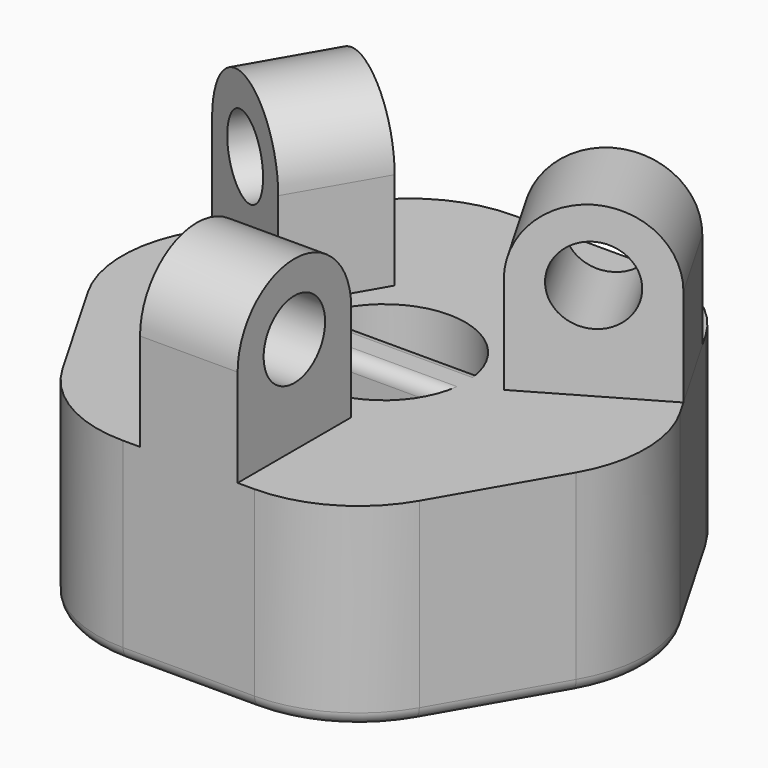
from build123d import *

# Parameters (mm, degrees)
F0_W            = 6.096
F0_H            = 1.778
F1_DEPTH        = 7.62
F2_R            = 1.5
F3_DEPTH        = 1.905
F3_COPIES_COUNT = 3
F4_R            = 5.08
F5_R            = 0.508


# Not quite as in the source:
# - a pattern or mirror of a feature is missing from the dataset's text; its kind, count and spacing are read off the source's solid


with BuildPart() as f1:
    # F0 (on Top) → F1 (new body)
    with BuildSketch(Plane.XY):
        Polygon((10.9985226281, 0), (5.499261314, 9.525), (-5.499261314, 9.525), (-10.9985226281, 0), (-5.499261314, -9.525), (5.499261314, -9.525), align=None)
        with BuildLine():
            ThreePointArc((3.048, 0.889), (3.1430896424, 0.4490128061), (3.175, 0))
            ThreePointArc((3.175, 0), (3.1430896424, -0.4490128061), (3.048, -0.889))
            ThreePointArc((3.048, -0.889), (0, -3.175), (-3.048, -0.889))
            ThreePointArc((-3.048, -0.889), (-3.175, 0), (-3.048, 0.889))
            ThreePointArc((-3.048, 0.889), (0, 3.175), (3.048, 0.889))
        make_face(mode=Mode.SUBTRACT)
        Rectangle(F0_W, F0_H)
        with BuildLine():
            Line((-3.048, -0.889), (-3.048, 0.889))
            ThreePointArc((-3.048, 0.889), (-3.175, 0), (-3.048, -0.889))
        make_face()
        with BuildLine():
            ThreePointArc((3.048, -0.889), (3.1430896424, -0.4490128061), (3.175, 0))
            ThreePointArc((3.175, 0), (3.1430896424, 0.4490128061), (3.048, 0.889))
            Line((3.048, 0.889), (3.048, -0.889))
        make_face()
    extrude(amount=F1_DEPTH)

    # F2 (on Right) → F3 (join, symmetric)
    with BuildSketch(Plane.YZ):
        with BuildLine():
            Line((-9.525, 7.62), (-3.985, 7.62))
            Line((-3.985, 7.62), (-3.985, 11.43))
            ThreePointArc((-3.985, 11.43), (-6.755, 14.2), (-9.525, 11.43))
            Line((-9.525, 11.43), (-9.525, 7.62))
        make_face()
        with Locations((-6.755, 11.43)):
            Circle(F2_R, mode=Mode.SUBTRACT)
    f3 = extrude(amount=F3_DEPTH, both=True)

    # F3_copies: F3 ×3 about axis
    f3_copies_axis = Axis((0, 0, 0), (0, 0, 1))
    for i in range(1, F3_COPIES_COUNT):
        add(f3.rotate(f3_copies_axis, i * 360 / F3_COPIES_COUNT))

    # F4
    f4_edges = [f1.edges().sort_by_distance(p)[0] for p in [
        (-5.499261, -9.525, 3.81),
        (-10.998523, 0, 3.81),
        (-5.499261, 9.525, 3.81),
        (5.499261, 9.525, 3.81),
        (10.998523, 0, 3.81),
        (5.499261, -9.525, 3.81),
    ]]
    fillet(f4_edges, radius=F4_R)

    # F5
    f5_edges = [f1.edges().sort_by_distance(p)[0] for p in [
        (0, -0.889, 7.62),
        (0, 0.889, 7.62),
        (0, -0.889, 0),
        (0, 0.889, 0),
        (0, 3.175, 0),
        (-8.248892, 4.7625, 0),
        (8.248892, 4.7625, 0),
        (10.212644, 0, 0),
        (5.106322, 8.844409, 0),
        (8.248892, -4.7625, 0),
        (0, 9.525, 0),
        (5.106322, -8.844409, 0),
        (-5.106322, 8.844409, 0),
        (0, -9.525, 0),
        (-5.106322, -8.844409, 0),
        (-10.212644, 0, 0),
        (-8.248892, -4.7625, 0),
        (0, -3.175, 0),
    ]]
    fillet(f5_edges, radius=F5_R)


solid = f1.part
